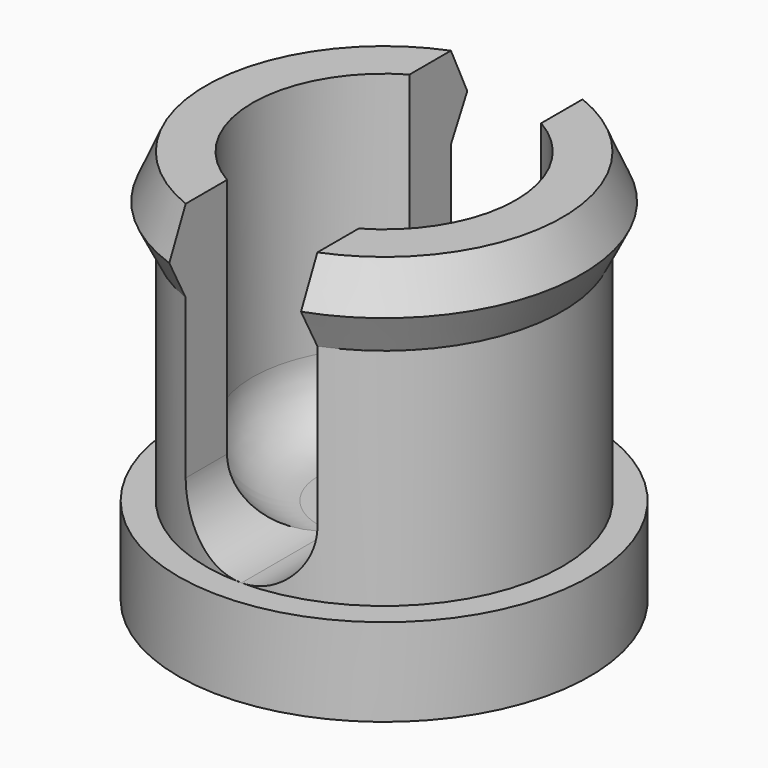
from build123d import *

# Parameters (mm, degrees)
F3_R     = 7.62
F4_DEPTH = 17.78
F6_DEPTH = 25.4
F7_R     = 3.80999


# Not quite as in the source:
# - a fillet or chamfer is up to 0.001 mm smaller than in the source, because OpenCascade refuses the exact size


with BuildPart() as f2:
    # F0 (on Front) → F2 (revolve)
    with BuildSketch(Plane.XZ):
        Polygon((-11.90625, 5.08), (-11.90625, 0), (0, 0), (0, 22.86), (-10.31875, 22.86), (-11.43, 20.32), (-10.31875, 18.0785163727), (-10.31875, 5.08), align=None)
    revolve(axis=Axis((0, 0, 7.382690208), (0, 0, 1)))

    # F3 (on face) → F4 (cut, through all)
    with BuildSketch(Plane.XY.offset(22.86)):
        Circle(F3_R)
    extrude(amount=-F4_DEPTH, mode=Mode.SUBTRACT)

    # F5 (on face) → F6 (cut)
    with BuildSketch(Plane.XY.offset(5.08)):
        Polygon((3.81, 14.0309315175), (-3.81, 14.0309315175), (-3.81, 3.81), (-3.81, -15.0898629799), (3.81, -15.0898629799), (3.81, 3.81), align=None)
    extrude(amount=F6_DEPTH, mode=Mode.SUBTRACT)

    # F7 (radius 3.81 in the source; OpenCascade refuses exactly that, so slightly less here)
    f7_edges = [f2.edges().sort_by_distance(p)[0] for p in [
        (-7.62, 0, 5.08),
        (7.62, 0, 5.08),
        (3.81, 8.094359, 5.08),
        (3.81, -8.094359, 5.08),
        (-3.81, -8.094359, 5.08),
        (-3.81, 8.094359, 5.08),
    ]]
    fillet(f7_edges, radius=F7_R)


solid = f2.part
